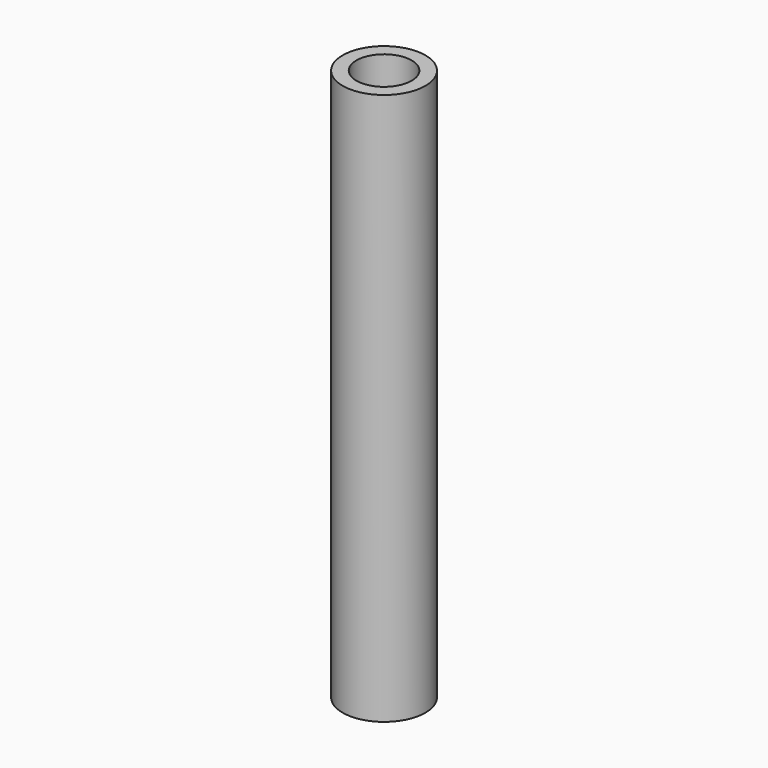
from build123d import *

# Parameters (mm, degrees)
F0_R     = 1.5
F0_R_2   = 1
F1_DEPTH = 20


# Not quite as in the source:
# - a feature names something its author has since deleted; it is built from what else it names


with BuildPart() as f1:
    # F0 (on Top) → F1 (new body)
    with BuildSketch(Plane.XY):
        Circle(F0_R)
        Circle(F0_R_2, mode=Mode.SUBTRACT)
    extrude(amount=F1_DEPTH)


solid = f1.part
